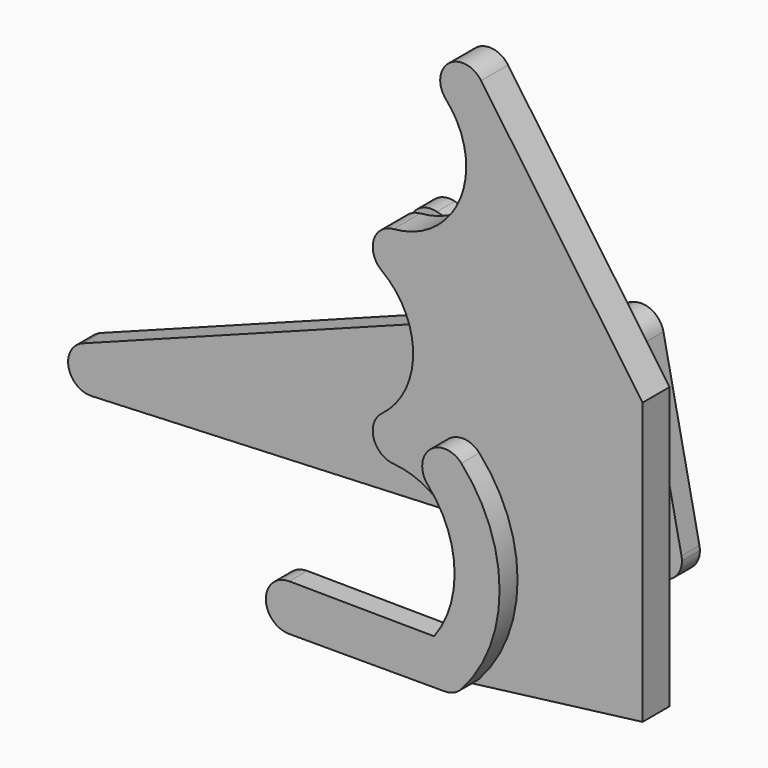
from build123d import *

# Parameters (mm, degrees)
F2_DEPTH  = 2
F4_DEPTH  = 2
F7_DEPTH  = 3
F10_DEPTH = 2
F12_DEPTH = 2


with BuildPart() as f2:
    # F1 (on Front) → F2 (new body)
    with BuildSketch(Plane.XZ):
        with BuildLine():
            ThreePointArc((-22.4976340457, 27.4567758947), (-20.7742896124, 27.8134864408), (-20, 29.3938769134))
            ThreePointArc((-20, 29.3938769134), (-20.4196095275, 30.619587301), (-21.5023659543, 31.3309779321))
            ThreePointArc((-21.5023659543, 31.3309779321), (-23.9371010187, 29.8915109591), (-22.4976340457, 27.4567758947))
        make_face()
        with BuildLine():
            ThreePointArc((-4.5031918506, 25.4128045476), (-4.9228013781, 26.6385149352), (-6.0055578049, 27.3499055663))
            ThreePointArc((-6.0055578049, 27.3499055663), (-8.4402928693, 25.9104385933), (-7.0008258964, 23.4757035289))
            ThreePointArc((-7.0008258964, 23.4757035289), (-5.277481463, 23.832414075), (-4.5031918506, 25.4128045476))
        make_face()
        with BuildLine():
            ThreePointArc((-21.5023659543, 31.3309779321), (-20.4196095275, 30.619587301), (-20, 29.3938769134))
            ThreePointArc((-20, 29.3938769134), (-20.7742896124, 27.8134864408), (-22.4976340457, 27.4567758947))
            Line((-22.4976340457, 27.4567758947), (-7.0008258964, 23.4757035289))
            ThreePointArc((-7.0008258964, 23.4757035289), (-8.4402928693, 25.9104385933), (-6.0055578049, 27.3499055663))
            Line((-6.0055578049, 27.3499055663), (-21.5023659543, 31.3309779321))
        make_face()
    extrude(amount=F2_DEPTH)


with BuildPart() as f4:
    # F3 (on Front) → F4 (new body)
    with BuildSketch(Plane.XZ):
        with BuildLine():
            ThreePointArc((-7.2077649929, 27.2845889067), (-7.6413600534, 23.7682459009), (-4.5031918506, 25.4128045476))
            ThreePointArc((-4.5031918506, 25.4128045476), (-4.5133195446, 25.6138224716), (-4.5436000564, 25.8128045476))
            ThreePointArc((-4.5436000564, 25.8128045476), (-5.5360800401, 27.1634315055), (-7.2077649929, 27.2845889067))
        make_face()
        with BuildLine():
            ThreePointArc((-4.5436000564, 25.8128045476), (-4.5133195446, 25.6138224716), (-4.5031918506, 25.4128045476))
            ThreePointArc((-4.5031918506, 25.4128045476), (-7.6413600534, 23.7682459009), (-7.2077649929, 27.2845889067))
            Line((-7.2077649929, 27.2845889067), (-54.5975598486, 9.4462217298))
            ThreePointArc((-54.5975598486, 9.4462217298), (-52.7548185036, 9.2189960173), (-51.8929867063, 7.5744373707))
            ThreePointArc((-51.8929867063, 7.5744373707), (-52.4489024417, 6.1907391967), (-53.8076073431, 5.5762606107))
            Line((-53.8076073431, 5.5762606107), (-3.2178124874, 7.7378934337))
            ThreePointArc((-3.2178124874, 7.7378934337), (-4.8790375607, 10.9676181215), (-1.3436000564, 10.1360701938))
            Line((-1.3436000564, 10.1360701938), (-4.5436000564, 25.8128045476))
        make_face()
        with BuildLine():
            ThreePointArc((-1.3031918506, 9.7360701938), (-1.3133195446, 9.9370881178), (-1.3436000564, 10.1360701938))
            ThreePointArc((-1.3436000564, 10.1360701938), (-4.8790375607, 10.9676181215), (-3.2178124874, 7.7378934337))
            ThreePointArc((-3.2178124874, 7.7378934337), (-1.859107586, 8.3523720198), (-1.3031918506, 9.7360701938))
        make_face()
        with BuildLine():
            ThreePointArc((-51.8929867063, 7.5744373707), (-52.7548185036, 9.2189960173), (-54.5975598486, 9.4462217298))
            ThreePointArc((-54.5975598486, 9.4462217298), (-55.8525785005, 7.1744373707), (-53.8076073431, 5.5762606107))
            ThreePointArc((-53.8076073431, 5.5762606107), (-52.4489024417, 6.1907391967), (-51.8929867063, 7.5744373707))
        make_face()
    extrude(amount=-F4_DEPTH)


with BuildPart() as f7:
    # F6 (on Front) → F7 (new body)
    with BuildSketch(Plane.XZ):
        with BuildLine():
            ThreePointArc((-15.75, -1.9843134833), (-14.5, -1.3228756555), (-14, 0))
            ThreePointArc((-14, 0), (-15.2827177269, 1.8669510279), (-17.4855061407, 1.339130877))
            ThreePointArc((-17.4855061407, 1.339130877), (-17.7728337373, -0.9257756424), (-15.75, -1.9843134833))
        make_face()
        with BuildLine():
            ThreePointArc((-17.4855061407, 1.339130877), (-15.2827177269, 1.8669510279), (-14, 0))
            ThreePointArc((-14, 0), (-14.5, -1.3228756555), (-15.75, -1.9843134833))
            Line((-15.75, -1.9843134833), (0, 0))
            Line((0, 0), (0, 25))
            Line((0, 25), (-14.3608981549, 45.5398896277))
            ThreePointArc((-14.3608981549, 45.5398896277), (-14.0923569922, 44.9946249095), (-14, 44.3938769134))
            ThreePointArc((-14, 44.3938769134), (-15.2827177269, 42.5269258855), (-17.4855061407, 43.0547460364))
            ThreePointArc((-17.4855061407, 43.0547460364), (-16.1854407971, 35.7680532322), (-22.1521728074, 31.3880793697))
            ThreePointArc((-22.1521728074, 31.3880793697), (-20.6406519237, 30.8609054773), (-20, 29.3938769134))
            ThreePointArc((-20, 29.3938769134), (-21.1060797511, 27.6047691501), (-23.2009065886, 27.7945572564))
            ThreePointArc((-23.2009065886, 27.7945572564), (-20.4040796488, 22.1969384567), (-23.2009065886, 16.599319657))
            ThreePointArc((-23.2009065886, 16.599319657), (-21.1060797511, 16.7891077633), (-20, 15))
            ThreePointArc((-20, 15), (-20.6406519237, 13.5329714361), (-22.1521728074, 13.0057975437))
            ThreePointArc((-22.1521728074, 13.0057975437), (-16.1854407971, 8.6258236812), (-17.4855061407, 1.339130877))
        make_face()
        with BuildLine():
            ThreePointArc((-23.2009065886, 16.599319657), (-23.9199104817, 14.4396931713), (-22.1521728074, 13.0057975437))
            ThreePointArc((-22.1521728074, 13.0057975437), (-20.6406519237, 13.5329714361), (-20, 15))
            ThreePointArc((-20, 15), (-21.1060797511, 16.7891077633), (-23.2009065886, 16.599319657))
        make_face()
        with BuildLine():
            ThreePointArc((-22.1521728074, 31.3880793697), (-23.9199104817, 29.9541837421), (-23.2009065886, 27.7945572564))
            ThreePointArc((-23.2009065886, 27.7945572564), (-21.1060797511, 27.6047691501), (-20, 29.3938769134))
            ThreePointArc((-20, 29.3938769134), (-20.6406519237, 30.8609054773), (-22.1521728074, 31.3880793697))
        make_face()
        with BuildLine():
            ThreePointArc((-14, 44.3938769134), (-14.0923569922, 44.9946249095), (-14.3608981549, 45.5398896277))
            ThreePointArc((-14.3608981549, 45.5398896277), (-17.2449428009, 45.9591620064), (-17.4855061407, 43.0547460364))
            ThreePointArc((-17.4855061407, 43.0547460364), (-15.2827177269, 42.5269258855), (-14, 44.3938769134))
        make_face()
    extrude(amount=F7_DEPTH)


with BuildPart() as f7_1:
    # F8: moved
    add(f7.part.moved(Location((0, -3, 0))))


with BuildPart() as f10:
    # F9 (on face) → F10 (new body)
    with BuildSketch(Plane.XZ.offset(6)):
        with BuildLine():
            ThreePointArc((-14.5144937322, -1.3391307361), (-14.133048938, -0.7172821845), (-14, 0))
            ThreePointArc((-14, 0), (-15.2827177269, 1.8669510279), (-17.4855061407, 1.339130877))
            ThreePointArc((-17.4855061407, 1.339130877), (-17.3391308066, -1.4855062043), (-14.5144937322, -1.3391307361))
        make_face()
        with BuildLine():
            ThreePointArc((-17.4855061407, 1.339130877), (-15.2827177269, 1.8669510279), (-14, 0))
            ThreePointArc((-14, 0), (-14.133048938, -0.7172821845), (-14.5144937322, -1.3391307361))
            ThreePointArc((-14.5144937322, -1.3391307361), (-11.1185016612, 7.5), (-14.5144937322, 16.3391307361))
            ThreePointArc((-14.5144937322, 16.3391307361), (-14.133048938, 15.7172821845), (-14, 15))
            ThreePointArc((-14, 15), (-15.2827178155, 13.133048938), (-17.4855062678, 13.6608692639))
            ThreePointArc((-17.4855062678, 13.6608692639), (-15.1185016612, 7.5000000949), (-17.4855061407, 1.339130877))
        make_face()
        with BuildLine():
            ThreePointArc((-14.5144937322, 16.3391307361), (-17.3391307361, 16.4855062678), (-17.4855062678, 13.6608692639))
            ThreePointArc((-17.4855062678, 13.6608692639), (-15.2827178155, 13.133048938), (-14, 15))
            ThreePointArc((-14, 15), (-14.133048938, 15.7172821845), (-14.5144937322, 16.3391307361))
        make_face()
    extrude(amount=F10_DEPTH)

    # F11 (on face) → F12 (join, through all)
    with BuildSketch(Plane.XZ.offset(8)):
        with BuildLine():
            Line((-29.8451329624, -2), (-16, -2))
            Line((-16, -2), (-15.9816370049, 1.9999156983))
            Line((-15.9816370049, 1.9999156983), (-29.8261863834, 2.1270347527))
            ThreePointArc((-29.8261863834, 2.1270347527), (-28.3792917586, 1.5160046749), (-27.7815720957, 0.0635608668))
            ThreePointArc((-27.7815720957, 0.0635608668), (-28.3859750802, -1.3955970155), (-29.8451329624, -2))
        make_face()
        with BuildLine():
            ThreePointArc((-29.8261863834, 2.1270347527), (-31.9086720839, 0.0730342561), (-29.8451329624, -2))
            ThreePointArc((-29.8451329624, -2), (-28.3859750802, -1.3955970155), (-27.7815720957, 0.0635608668))
            ThreePointArc((-27.7815720957, 0.0635608668), (-28.3792917586, 1.5160046749), (-29.8261863834, 2.1270347527))
        make_face()
    extrude(amount=-F12_DEPTH)


solid = Compound([f2.part, f4.part, f7_1.part, f10.part])
